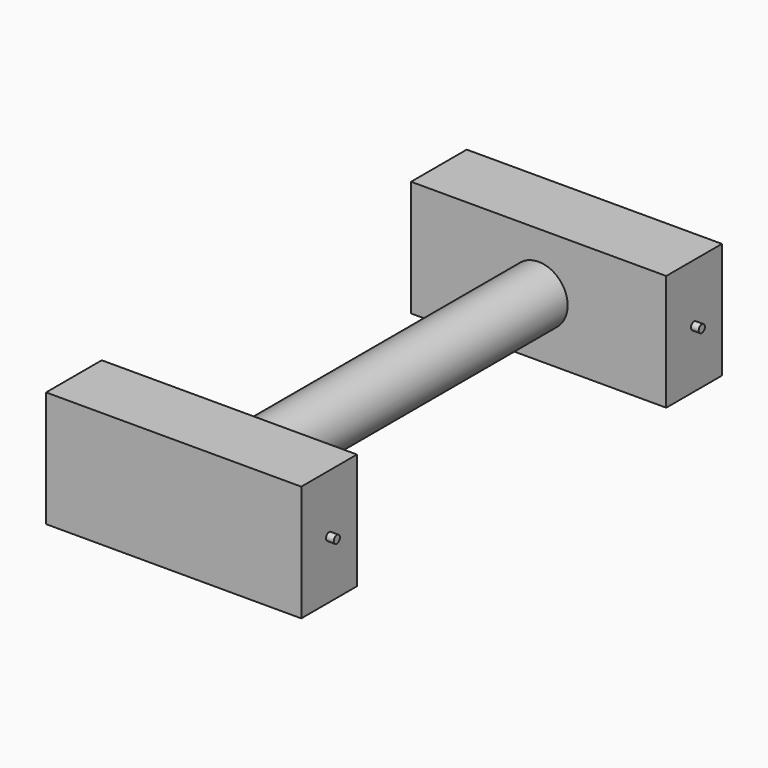
from build123d import *

# Parameters (mm, degrees)
F0_W     = 66
F0_H     = 30
F0_R     = 7.5
F1_DEPTH = 18
F3_R     = 1
F4_DEPTH = 70
F5_DEPTH = 100
F6_W     = 66
F6_H     = 30
F6_R     = 7.5
F7_DEPTH = 18
F8_R     = 1
F9_DEPTH = 70


# Not quite as in the source:
# - a feature names something its author has since deleted; it is built from what else it names


with BuildPart() as f1:
    # F0 (on Front) → F1 (new body)
    with BuildSketch(Plane.XZ):
        Rectangle(F0_W, F0_H)
        Circle(F0_R, mode=Mode.SUBTRACT)
        Circle(F0_R)
    extrude(amount=F1_DEPTH)

    # F3 (on offset) → F4 (join)
    with BuildSketch(Plane.YZ.offset(35)):
        with Locations((-9.0000117198, 0)):
            Circle(F3_R)
    extrude(amount=-F4_DEPTH)

    # F0 (on Front) → F5 (join)
    with BuildSketch(Plane.XZ):
        Circle(F0_R)
    extrude(amount=-F5_DEPTH)

    # F6 (on face) → F7 (join)
    with BuildSketch(Plane(origin=(0, 100, 0), x_dir=(-1, 0, 0), z_dir=(0, 1, 0))):
        Rectangle(F6_W, F6_H)
        Circle(F6_R, mode=Mode.SUBTRACT)
        Circle(F6_R)
    extrude(amount=F7_DEPTH)

    # F8 (on offset) → F9 (join)
    with BuildSketch(Plane.YZ.offset(35)):
        with Locations((109, 0)):
            Circle(F8_R)
    extrude(amount=-F9_DEPTH)


solid = f1.part
